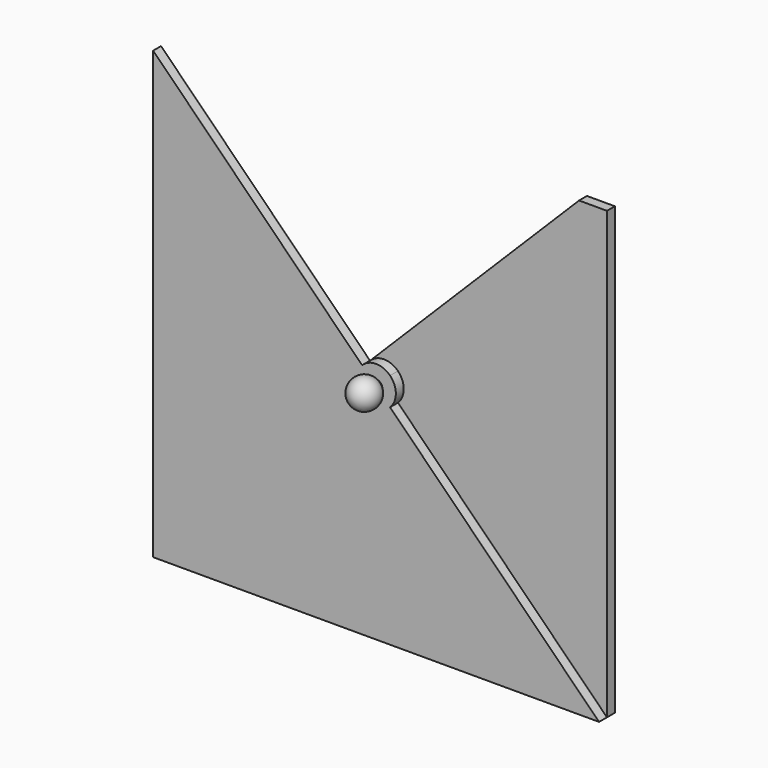
from build123d import *

# Parameters (mm, degrees)
F0_R      = 2.032
F1_DEPTH  = 3.175
F4_ANGLE  = 90
F6_R      = 6.35
F7_DEPTH  = 6.35
F9_DEPTH  = 3.175
F13_ANGLE = 180
F16_DEPTH = 3.176


# Not quite as in the source:
# - a feature of the source that left no trace in its solid (it failed there, or was rolled back) is left out


with BuildPart() as f1:
    # F0 (on Front) → F1 (new body)
    with BuildSketch(Plane.XZ):
        Polygon((76.2, 76.2), (-76.2, -76.2), (76.2, -76.2), align=None)
        with Locations((4.4901280605, -4.4901280605)):
            Circle(F0_R, mode=Mode.SUBTRACT)
    extrude(amount=F1_DEPTH)


with BuildPart() as f4_1:
    # F4: copy of F1
    add(f1.part.rotate(Axis((4.4901280605, -59.5605373383, -4.4901280605), (0, -1, 0)), F4_ANGLE))


with BuildPart() as f4_1_1:
    # F5: moved
    add(f4_1.part.moved(Location((0, -3.175, 0))))

    # F8 (on face) → F9 (cut, through all)
    with BuildSketch(Plane.XZ.offset(6.35)):
        with BuildLine():
            ThreePointArc((8.9802561211, -8.9802561211), (4.4901280539, -10.8401280605), (-9.4e-09, -8.9802561117))
            Line((-9.4e-09, -8.9802561117), (76.2, -85.1802561211))
            Line((76.2, -85.1802561211), (76.2, -76.2))
            Line((76.2, -76.2), (8.9802561211, -8.9802561211))
        make_face()
        with BuildLine():
            ThreePointArc((-9.4e-09, -8.9802561117), (-1.8598719395, -4.4901280539), (0, 0))
            Line((0, 0), (-67.2197438789, 67.2197438789))
            Line((-67.2197438789, 67.2197438789), (-76.2, 67.2197438789))
            Line((-76.2, 67.2197438789), (-9.4e-09, -8.9802561117))
        make_face()
    extrude(amount=-F9_DEPTH, mode=Mode.SUBTRACT)


with BuildPart() as f7:
    # F6 (on face) → F7 (new body)
    with BuildSketch(Plane.XZ.offset(6.35)):
        with Locations((4.4901280605, -4.4901280605)):
            Circle(F6_R)
    extrude(amount=F7_DEPTH)


with BuildPart() as f4_1_2:
    # F13: moved
    add(f4_1_1.part.rotate(Axis((4.4901280605, -59.5605373383, -4.4901280605), (0, -1, 0)), F13_ANGLE))


with BuildPart() as f1_1:
    add(f1.part)

    # F15 (on face) → F16 (cut, through all)
    with BuildSketch(Plane.XZ.offset(3.175)):
        Polygon((-76.2, -76.2), (-67.2197438789, -76.2), (-67.2197438789, -67.2197438789), align=None)
        Polygon((67.2197438789, 67.2197438789), (76.2, 67.2197438789), (76.2, 76.2), align=None)
    extrude(amount=-F16_DEPTH, mode=Mode.SUBTRACT)


with BuildPart() as f19:
    # F18 (on face) → F19 (revolve)
    with BuildSketch(Plane(origin=(0, 0, 0), x_dir=(0.7071067812, 0, -0.7071067812), z_dir=(0.7071067812, 0, 0.7071067812))):
        with BuildLine():
            Line((6.35, -6.35), (6.35, -15.875))
            ThreePointArc((6.35, -15.875), (11.1125, -11.1125), (6.35, -6.35))
        make_face()
    revolve(axis=Axis((4.4901280605, -17.9845464677, -4.4901280605), (0, -1, 0)))


solid = Compound([f4_1_2.part, f1_1.part, f19.part])
